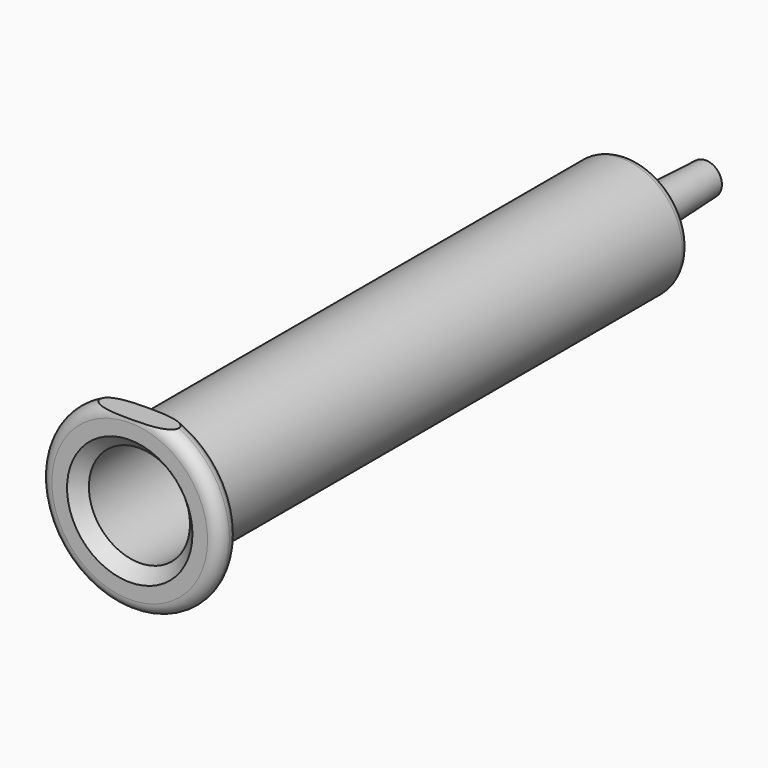
from build123d import *

# Parameters (mm, degrees)
F0_R      = 7.5
F0_R_2    = 6.25
F1_DEPTH  = 77
F2_R      = 11.125
F2_R_2    = 7.5
F2_R_3    = 6.25
F3_DEPTH  = 3
F4_R      = 1.49999
F6_DEPTH  = 25
F7_SIZE   = 1.5
F8_R      = 7.5
F9_DEPTH  = 1.5
F10_R     = 1
F13_R     = 0.5
F14_R     = 2
F15_DEPTH = 25
F16_R     = 0.5


# Not quite as in the source:
# - a fillet or chamfer is up to 0.001 mm smaller than in the source, because OpenCascade refuses the exact size


with BuildPart() as f1:
    # F0 (on Front) → F1 (new body)
    with BuildSketch(Plane.XZ):
        Circle(F0_R)
        Circle(F0_R_2, mode=Mode.SUBTRACT)
    extrude(amount=F1_DEPTH)

    # F2 (on face) → F3 (join)
    with BuildSketch(Plane.XZ.offset(77)):
        Circle(F2_R)
        Circle(F2_R_2, mode=Mode.SUBTRACT)
        Circle(F2_R_2)
        Circle(F2_R_3, mode=Mode.SUBTRACT)
    extrude(amount=-F3_DEPTH)

    # F4 (radius 1.5 in the source; OpenCascade refuses exactly that, so slightly less here)
    f4_edges = [f1.edges().sort_by_distance(p)[0] for p in [
        (-11.125, -77, 0),
        (-11.125, -74, 0),
    ]]
    fillet(f4_edges, radius=F4_R)

    # F5 (on face) → F6 (cut)
    with BuildSketch(Plane.XZ.offset(77)):
        Polygon((-7.5801494531, 15.4223963618), (-10.2109283504, 10), (17.5064372194, 10), (14.5523855463, 16.5495146066), align=None)
    extrude(amount=-F6_DEPTH, mode=Mode.SUBTRACT)

    # F7
    f7_edges = [f1.edges().sort_by_distance(p)[0] for p in [
        (-6.25, -77, 0),
    ]]
    chamfer(f7_edges, length=F7_SIZE)

    # F8 (on face) → F9 (join)
    with BuildSketch(Plane(origin=(0, 0, 0), x_dir=(-1, 0, 0), z_dir=(0, 1, 0))):
        Circle(F8_R)
    extrude(amount=-F9_DEPTH)

    # F10
    f10_edges = [f1.edges().sort_by_distance(p)[0] for p in [
        (-7.5, 0, 0),
    ]]
    fillet(f10_edges, radius=F10_R)

    # F11 (on Right) → F12 (revolve)
    with BuildSketch(Plane.YZ):
        Polygon((0, -2), (0, -2.5), (12, -2), (12, -1.5), align=None)
    revolve(axis=Axis((0, 5.0854310393, 0), (0, -1, 0)))

    # F13
    f13_edges = [f1.edges().sort_by_distance(p)[0] for p in [
        (0, 0, 2.5),
    ]]
    fillet(f13_edges, radius=F13_R)

    # F14 (on face) → F15 (cut)
    with BuildSketch(Plane(origin=(0, 0, 0), x_dir=(-1, 0, 0), z_dir=(0, 1, 0))):
        Circle(F14_R)
    extrude(amount=-F15_DEPTH, mode=Mode.SUBTRACT)

    # F16
    f16_edges = [f1.edges().sort_by_distance(p)[0] for p in [
        (2, -1.5, 0),
    ]]
    fillet(f16_edges, radius=F16_R)


solid = f1.part
